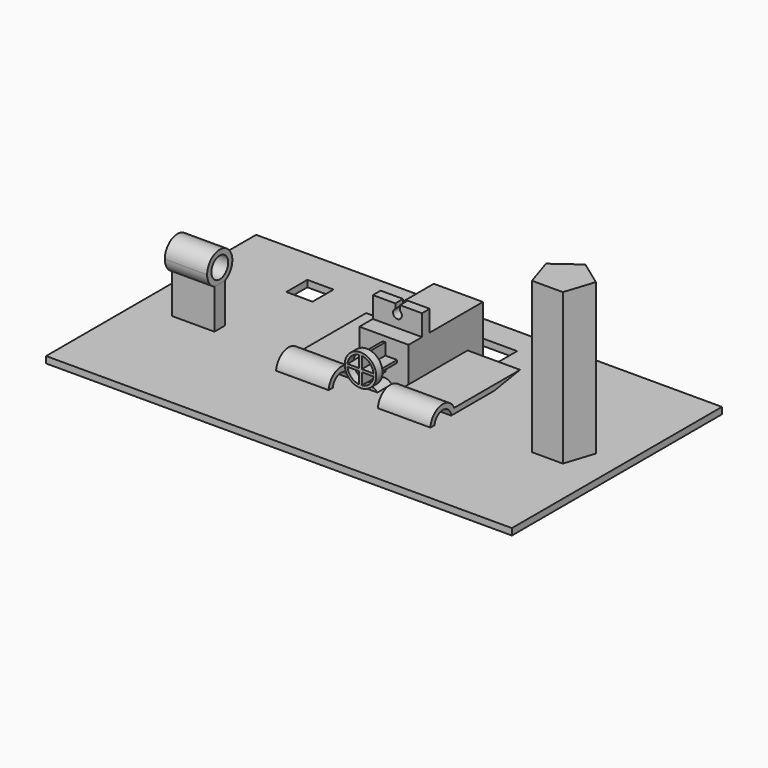
from build123d import *

# Parameters (mm, degrees)
F0_W      = 112.6744
F0_H      = 63.5
F0_W_2    = 10.2123171091
F0_H_2    = 3.1538007315
F0_W_3    = 6.35
F0_H_3    = 6.35
F1_DEPTH  = 1.5875
F2_DEPTH  = 38.1
F3_R      = 2.2987
F4_DEPTH  = 4.318
F5_DEPTH  = 6.7564
F6_DEPTH  = 22.479
F7_W      = 11.8872
F7_H      = 2.3368
F8_DEPTH  = 5.08
F10_DEPTH = 2.48331
F11_W     = 11.8872
F11_H     = 2.3368
F12_DEPTH = 5.08
F14_DEPTH = 25.4
F15_R     = 1.016
F16_DEPTH = 25.4
F18_DEPTH = 7.112
F19_R     = 3.81
F19_R_2   = 3.1623
F20_DEPTH = 1.905
F21_R     = 5.2705
F21_R_2   = 2.413
F22_DEPTH = 1.60334
F23_R     = 2.54
F24_DEPTH = 12.7
F25_R     = 2.5415511009
F26_DEPTH = 12.7
F27_DEPTH = 11.176
F28_R     = 2.54
F29_DEPTH = 10.24225


with BuildPart() as f1:
    # F0 (on Top) → F1 (new body)
    with BuildSketch(Plane.XY):
        Rectangle(F0_W, F0_H)
        with Locations((-42.8348071873, -2.54)):
            Rectangle(F0_W_2, F0_H_2, mode=Mode.SUBTRACT)
        with Locations((-34.0979072105, 20.228437902)):
            Rectangle(F0_W_3, F0_H_3, mode=Mode.SUBTRACT)
        Polygon((0, 2.921), (0, 25.4), (5.9436, 25.4), (11.8872, 25.4), (11.8872, 2.921), (5.9436, 2.921), align=None, mode=Mode.SUBTRACT)
        Polygon((49.6764088785, 1.9622579143), (47.3696363521, -5.1372579143), (39.9047636479, -5.1372579143), (37.5979911215, 1.9622579143), (43.6372, 6.35), align=None, mode=Mode.SUBTRACT)
    extrude(amount=F1_DEPTH)

    # F0 (on Top) → F2 (join)
    with BuildSketch(Plane.XY):
        Polygon((39.9047636479, -5.1372579143), (47.3696363521, -5.1372579143), (49.6764088785, 1.9622579143), (43.6372, 6.35), (37.5979911215, 1.9622579143), align=None)
    extrude(amount=F2_DEPTH)

    # F0 (on Top) → F27 (join)
    with BuildSketch(Plane.XY):
        with Locations((-42.8348071873, -2.54)):
            Rectangle(F0_W_2, F0_H_2)
    extrude(amount=F27_DEPTH)

    # F28 (on face) → F29 (join)
    with BuildSketch(Plane(origin=(-47.9409657419, 0, 0), x_dir=(0, -1, 0), z_dir=(-1, 0, 0))):
        with BuildLine():
            ThreePointArc((4.1169003658, 11.176), (5.7434427101, 12.5818188188), (6.35, 14.6443548314))
            ThreePointArc((6.35, 14.6443548314), (0.4774639874, 17.8477975415), (0.9630996342, 11.176))
            Line((0.9630996342, 11.176), (4.1169003658, 11.176))
        make_face()
        with Locations((2.54, 14.6443548314)):
            Circle(F28_R, mode=Mode.SUBTRACT)
    extrude(amount=-F29_DEPTH)


with BuildPart() as f4:
    # F3 (on Front) → F4 (new body)
    with BuildSketch(Plane.XZ):
        with BuildLine():
            ThreePointArc((0, -11.3157), (4.2027598647, -9.5748598647), (5.9436, -5.3721))
            ThreePointArc((5.9436, -5.3721), (4.9946233933, -2.1502809302), (2.4507276268, 0.0427236407))
            ThreePointArc((2.4507276268, 0.0427236407), (2.4510069049, 0.0213626317), (2.4511, 0))
            ThreePointArc((2.4511, 0), (-0.0213626317, -2.4510069049), (-2.4507276268, 0.0427236407))
            ThreePointArc((-2.4507276268, 0.0427236407), (-4.9946233933, -2.1502809302), (-5.9436, -5.3721))
            ThreePointArc((-5.9436, -5.3721), (-4.2027598647, -9.5748598647), (0, -11.3157))
        make_face()
        with Locations((0, -5.3721)):
            Circle(F3_R, mode=Mode.SUBTRACT)
        with Locations((0, -5.3721)):
            Circle(F3_R)
        with BuildLine():
            ThreePointArc((2.4511, 0), (2.4510069049, 0.0213626317), (2.4507276268, 0.0427236407))
            ThreePointArc((2.4507276268, 0.0427236407), (0, 0.5715), (-2.4507276268, 0.0427236407))
            ThreePointArc((-2.4507276268, 0.0427236407), (-0.0213626317, -2.4510069049), (2.4511, 0))
        make_face()
        with BuildLine():
            ThreePointArc((-2.4507276268, 0.0427236407), (0, 0.5715), (2.4507276268, 0.0427236407))
            ThreePointArc((2.4507276268, 0.0427236407), (0, 2.4511), (-2.4507276268, 0.0427236407))
        make_face()
    extrude(amount=F4_DEPTH)

    # F3 (on Front) → F5 (join)
    with BuildSketch(Plane.XZ):
        with Locations((0, -5.3721)):
            Circle(F3_R)
    extrude(amount=F5_DEPTH)

    # F3 (on Front) → F6 (join)
    with BuildSketch(Plane.XZ):
        with BuildLine():
            ThreePointArc((2.4511, 0), (2.4510069049, 0.0213626317), (2.4507276268, 0.0427236407))
            ThreePointArc((2.4507276268, 0.0427236407), (0, 0.5715), (-2.4507276268, 0.0427236407))
            ThreePointArc((-2.4507276268, 0.0427236407), (-0.0213626317, -2.4510069049), (2.4511, 0))
        make_face()
        with BuildLine():
            ThreePointArc((0, -11.3157), (4.2027598647, -9.5748598647), (5.9436, -5.3721))
            ThreePointArc((5.9436, -5.3721), (4.9946233933, -2.1502809302), (2.4507276268, 0.0427236407))
            ThreePointArc((2.4507276268, 0.0427236407), (2.4510069049, 0.0213626317), (2.4511, 0))
            ThreePointArc((2.4511, 0), (-0.0213626317, -2.4510069049), (-2.4507276268, 0.0427236407))
            ThreePointArc((-2.4507276268, 0.0427236407), (-4.9946233933, -2.1502809302), (-5.9436, -5.3721))
            ThreePointArc((-5.9436, -5.3721), (-4.2027598647, -9.5748598647), (0, -11.3157))
        make_face()
        with Locations((0, -5.3721)):
            Circle(F3_R, mode=Mode.SUBTRACT)
        with Locations((0, -5.3721)):
            Circle(F3_R)
        with BuildLine():
            Line((5.9436, -11.3157), (5.9436, -5.3721))
            ThreePointArc((5.9436, -5.3721), (4.2027598647, -9.5748598647), (0, -11.3157))
            Line((0, -11.3157), (5.9436, -11.3157))
        make_face()
        with BuildLine():
            ThreePointArc((0, -11.3157), (-4.2027598647, -9.5748598647), (-5.9436, -5.3721))
            Line((-5.9436, -5.3721), (-5.9436, -11.3157))
            Line((-5.9436, -11.3157), (0, -11.3157))
        make_face()
        with BuildLine():
            Line((5.9436, -5.3721), (5.9436, 11.3157))
            Line((5.9436, 11.3157), (-5.9436, 11.3157))
            Line((-5.9436, 11.3157), (-5.9436, -5.3721))
            ThreePointArc((-5.9436, -5.3721), (-4.9946233933, -2.1502809302), (-2.4507276268, 0.0427236407))
            ThreePointArc((-2.4507276268, 0.0427236407), (0, 2.4511), (2.4507276268, 0.0427236407))
            ThreePointArc((2.4507276268, 0.0427236407), (4.9946233933, -2.1502809302), (5.9436, -5.3721))
        make_face()
        with BuildLine():
            ThreePointArc((-2.4507276268, 0.0427236407), (0, 0.5715), (2.4507276268, 0.0427236407))
            ThreePointArc((2.4507276268, 0.0427236407), (0, 2.4511), (-2.4507276268, 0.0427236407))
        make_face()
    extrude(amount=-F6_DEPTH)

    # F7 (on face) → F8 (join)
    with BuildSketch(Plane.XY.offset(11.3157)):
        with Locations((0, 5.2308826215)):
            Rectangle(F7_W, F7_H)
    extrude(amount=F8_DEPTH)

    # F9 (on face) → F10 (cut)
    with BuildSketch(Plane.XZ.offset(-4.0624826215)):
        with BuildLine():
            ThreePointArc((-0.5192814278, 15.2193846703), (-0.5404131812, 13.3677088098), (1.0668, 14.2875))
            ThreePointArc((1.0668, 14.2875), (0.9495907573, 14.7736477487), (0.6237185722, 15.152969458))
            Line((0.6237185722, 15.152969458), (0.6237185722, 15.0088137016))
            Line((0.6237185722, 15.0088137016), (-0.5192814278, 15.0088137016))
            Line((-0.5192814278, 15.0088137016), (-0.5192814278, 15.2193846703))
        make_face()
        with BuildLine():
            Line((0.6237185722, 15.0088137016), (0.6237185722, 15.152969458))
            ThreePointArc((0.6237185722, 15.152969458), (0.061883151, 15.3525036223), (-0.5192814278, 15.2193846703))
            Line((-0.5192814278, 15.2193846703), (-0.5192814278, 15.0088137016))
            Line((-0.5192814278, 15.0088137016), (0.6237185722, 15.0088137016))
        make_face()
        with BuildLine():
            ThreePointArc((-0.5192814278, 15.2193846703), (0.061883151, 15.3525036223), (0.6237185722, 15.152969458))
            Line((0.6237185722, 15.152969458), (0.6237185722, 16.3957))
            Line((0.6237185722, 16.3957), (-0.5192814278, 16.3957))
            Line((-0.5192814278, 16.3957), (-0.5192814278, 15.2193846703))
        make_face()
    extrude(amount=-F10_DEPTH, mode=Mode.SUBTRACT)

    # F11 (on face) → F12 (join)
    with BuildSketch(Plane(origin=(0, 0, -11.3157), x_dir=(1, 0, 0), z_dir=(0, 0, -1))):
        with Locations((0, -5.22986)):
            Rectangle(F11_W, F11_H)
    extrude(amount=F12_DEPTH)

    # F13 (on face) → F14 (cut)
    with BuildSketch(Plane.XZ.offset(-4.06146)):
        with BuildLine():
            Line((-0.62484, -16.3957), (0.51816, -16.3957))
            Line((0.51816, -16.3957), (0.51816, -15.2200086886))
            ThreePointArc((0.51816, -15.2200086886), (0.0632140085, -13.2225745429), (-0.62484, -15.1521601728))
            Line((-0.62484, -15.1521601728), (-0.62484, -16.3957))
        make_face()
    extrude(amount=-F14_DEPTH, mode=Mode.SUBTRACT)

    # F15 (on face) → F16 (cut)
    with BuildSketch(Plane.XZ.offset(6.7564)):
        with Locations((0, -5.3721)):
            Circle(F15_R)
    extrude(amount=-F16_DEPTH, mode=Mode.SUBTRACT)


with BuildPart() as f18:
    # F17 (on face) → F18 (new body)
    with BuildSketch(Plane.XZ):
        Polygon((0.3175, 10.0457), (0, 10.0457), (-0.3175, 10.0457), (-0.3175, 7.2009), (-3.1623, 7.2009), (-3.1623, 6.8834), (-3.1623, 6.5659), (-0.3175, 6.5659), (-0.3175, 3.7211), (0.3175, 3.7211), (0.3175, 6.5659), (3.1623, 6.5659), (3.1623, 7.2009), (0.3175, 7.2009), align=None)
    extrude(amount=F18_DEPTH)


with BuildPart() as f20:
    # F19 (on face) → F20 (new body)
    with BuildSketch(Plane.XZ.offset(7.112)):
        with Locations((0, 6.8834)):
            Circle(F19_R)
        with Locations((0, 6.8834)):
            Circle(F19_R_2, mode=Mode.SUBTRACT)
    extrude(amount=-F20_DEPTH)


with BuildPart() as f22:
    # F21 (on face) → F22 (new body)
    with BuildSketch(Plane.XZ.offset(6.7564)):
        with Locations((0, -5.3721)):
            Circle(F21_R)
        with Locations((0, -5.3721)):
            Circle(F21_R_2, mode=Mode.SUBTRACT)
    extrude(amount=-F22_DEPTH)


with BuildPart() as f24:
    # F23 (on face) → F24 (new body)
    with BuildSketch(Plane(origin=(-5.9436, 0, 0), x_dir=(0, -1, 0), z_dir=(-1, 0, 0))):
        with BuildLine():
            Line((2.0627967482, 2.8112942947), (-17.8912921724, 2.8112942947))
            Line((-17.8912921724, 2.8112942947), (2.0627967482, -0.3275605978))
            ThreePointArc((2.0627967482, -0.3275605978), (1.7245394649, 1.2418668484), (2.0627967482, 2.8112942947))
        make_face()
        with BuildLine():
            ThreePointArc((9.3445394649, 1.2418668484), (6.3372723748, 4.9663426337), (2.0627967482, 2.8112942947))
            ThreePointArc((2.0627967482, 2.8112942947), (1.7245394649, 1.2418668484), (2.0627967482, -0.3275605978))
            ThreePointArc((2.0627967482, -0.3275605978), (6.3372723748, -2.4826089369), (9.3445394649, 1.2418668484))
        make_face()
        with Locations((5.5345394649, 1.2418668484)):
            Circle(F23_R, mode=Mode.SUBTRACT)
    extrude(amount=F24_DEPTH)


with BuildPart() as f26:
    # F25 (on face) → F26 (new body)
    with BuildSketch(Plane.YZ.offset(5.9436)):
        with BuildLine():
            ThreePointArc((-2.1123207355, -0.3903365839), (-1.8202639704, 0.4250587769), (-1.7211828816, 1.2854945307))
            ThreePointArc((-1.7211828816, 1.2854945307), (-1.8098288556, 2.0999280003), (-2.0716152208, 2.8762191082))
            ThreePointArc((-2.0716152208, 2.8762191082), (-9.2921294544, 1.3326645995), (-2.1123207355, -0.3903365839))
        make_face()
        with Locations((-5.5068031124, 1.2854945307)):
            Circle(F25_R, mode=Mode.SUBTRACT)
        with BuildLine():
            ThreePointArc((-2.0716152208, 2.8762191082), (-1.8098288556, 2.0999280003), (-1.7211828816, 1.2854945307))
            ThreePointArc((-1.7211828816, 1.2854945307), (-1.8202639704, 0.4250587769), (-2.1123207355, -0.3903365839))
            Line((-2.1123207355, -0.3903365839), (17.8405269985, 2.8762191082))
            Line((17.8405269985, 2.8762191082), (-2.0716152208, 2.8762191082))
        make_face()
    extrude(amount=F26_DEPTH)


solid = Compound([f1.part, f4.part, f18.part, f20.part, f22.part, f24.part, f26.part])
